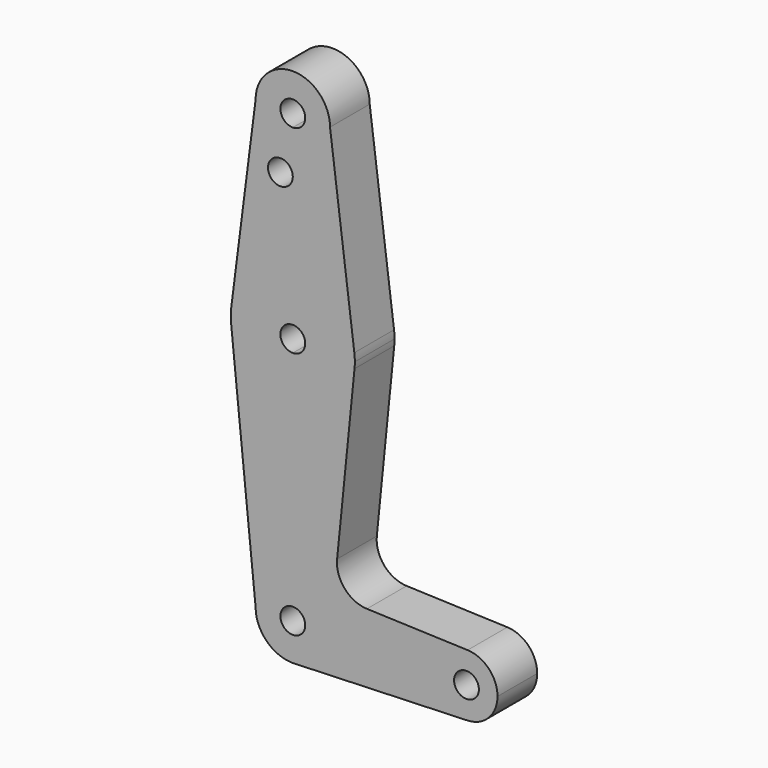
from build123d import *

# Parameters (mm, degrees)
F0_R     = 3.175
F1_DEPTH = 12.7


# Not quite as in the source:
# - a feature names something its author has since deleted; it is built from what else it names


with BuildPart() as f1:
    # F0 (on Front) → F1 (new body)
    with BuildSketch(Plane.XZ):
        with BuildLine():
            Line((0, 9.525), (0, 3.175))
            ThreePointArc((0, 3.175), (2.2450640303, 2.2450640303), (3.175, 0))
            Line((3.175, 0), (9.525, 0))
            ThreePointArc((9.525, 0), (6.7351920908, 6.7351920908), (0, 9.525))
        make_face()
        with BuildLine():
            ThreePointArc((3.175, 0), (-2.2450640303, -2.2450640303), (0, 3.175))
            Line((0, 3.175), (0, 9.525))
            ThreePointArc((0, 9.525), (-6.7351920908, 6.7351920908), (-9.525, 0))
            ThreePointArc((-9.525, 0), (-6.7351920908, -6.7351920908), (0, -9.525))
            Line((0, -9.525), (0.6773435479, -9.500885786))
            ThreePointArc((0.6773435479, -9.500885786), (6.9705567315, -6.4912990883), (9.525, 0))
            Line((9.525, 0), (3.175, 0))
        make_face()
        with BuildLine():
            ThreePointArc((-9.525, 0), (-6.7351920908, 6.7351920908), (0, 9.525))
            Line((0, 9.525), (0, 47.625))
            ThreePointArc((0, 47.625), (-10.644756084, 51.722700101), (-15.7942028036, 61.9003804205))
            Line((-15.7942028036, 61.9003804205), (-9.525, 0))
        make_face()
        with BuildLine():
            Line((0, 47.625), (0, 9.525))
            ThreePointArc((0, 9.525), (6.7351920908, 6.7351920908), (9.525, 0))
            Line((9.525, 0), (36.5125, 0))
            ThreePointArc((36.5125, 0), (38.9384772185, 5.7120069047), (44.7334821429, 7.9324362036))
            Line((44.7334821429, 7.9324362036), (18.9676000005, 8.8532337108))
            ThreePointArc((18.9676000005, 8.8532337108), (13.2611998974, 11.5713591498), (11.3411865923, 17.5933818124))
            Line((11.3411865923, 17.5933818124), (15.7954255641, 61.9125))
            ThreePointArc((15.7954255641, 61.9125), (10.6492737428, 51.7267849017), (0, 47.625))
        make_face()
        with BuildLine():
            Line((36.5125, 0), (9.525, 0))
            ThreePointArc((9.525, 0), (6.9705567315, -6.4912990883), (0.6773435479, -9.500885786))
            Line((0.6773435479, -9.500885786), (44.7324052746, -7.9324746146))
            ThreePointArc((44.7324052746, -7.9324746146), (38.9380895153, -5.7116327839), (36.5125, 0))
        make_face()
        with BuildLine():
            ThreePointArc((44.7334821429, 7.9324362036), (38.9384772185, 5.7120069047), (36.5125, 0))
            ThreePointArc((36.5125, 0), (38.9380895153, -5.7116327839), (44.7324052746, -7.9324746146))
            ThreePointArc((44.7324052746, -7.9324746146), (50.1616327839, -5.5119104847), (52.3875, 0))
            ThreePointArc((52.3875, 0), (50.1620069047, 5.5115227815), (44.7334821429, 7.9324362036))
        make_face()
        with BuildLine():
            ThreePointArc((47.625, 0), (44.45, -3.175), (41.275, 0))
            ThreePointArc((41.275, 0), (44.45, 3.175), (47.625, 0))
        make_face(mode=Mode.SUBTRACT)
        with BuildLine():
            Line((0, 60.325), (0, 47.625))
            ThreePointArc((0, 47.625), (10.6492737428, 51.7267849017), (15.7954255641, 61.9125))
            ThreePointArc((15.7954255641, 61.9125), (15.8550939106, 62.7052534459), (15.875, 63.5))
            ThreePointArc((15.875, 63.5), (15.8430821396, 64.5061676396), (15.7474569047, 65.5082893304))
            ThreePointArc((15.7474569047, 65.5082893304), (10.4912828548, 75.4142187767), (0, 79.375))
            Line((0, 79.375), (0, 66.675))
            ThreePointArc((0, 66.675), (2.2450640303, 65.7450640303), (3.175, 63.5))
            ThreePointArc((3.175, 63.5), (2.2450640303, 61.2549359697), (0, 60.325))
        make_face()
        with BuildLine():
            ThreePointArc((-15.7942028036, 61.9003804205), (-10.644756084, 51.722700101), (0, 47.625))
            Line((0, 47.625), (0, 60.325))
            ThreePointArc((0, 60.325), (-3.175, 63.5), (0, 66.675))
            Line((0, 66.675), (0, 79.375))
            ThreePointArc((0, 79.375), (-10.4912828548, 75.4142187767), (-15.7474569047, 65.5082893304))
            ThreePointArc((-15.7474569047, 65.5082893304), (-15.873667691, 63.7056672947), (-15.7942028036, 61.9003804205))
        make_face()
        with BuildLine():
            Line((0, 100.0252), (0, 79.375))
            ThreePointArc((0, 79.375), (10.4912828548, 75.4142187767), (15.7474569047, 65.5082893304))
            Line((15.7474569047, 65.5082893304), (9.525, 114.3))
            ThreePointArc((9.525, 114.3), (6.7351920908, 107.5648079092), (0, 104.775))
            Line((0, 104.775), (0, 100.0252))
        make_face()
        with BuildLine():
            Line((-9.525, 114.3), (-15.7474569047, 65.5082893304))
            ThreePointArc((-15.7474569047, 65.5082893304), (-10.4912828548, 75.4142187767), (0, 79.375))
            Line((0, 79.375), (0, 100.0252))
            Line((0, 100.0252), (0, 104.775))
            ThreePointArc((0, 104.775), (-6.7351920908, 107.5648079092), (-9.525, 114.3))
        make_face()
        with Locations((-3.175, 100.0252)):
            Circle(F0_R, mode=Mode.SUBTRACT)
        with BuildLine():
            ThreePointArc((9.525, 114.3), (0, 123.825), (-9.525, 114.3))
            ThreePointArc((-9.525, 114.3), (-6.7351920908, 107.5648079092), (0, 104.775))
            ThreePointArc((0, 104.775), (6.7351920908, 107.5648079092), (9.525, 114.3))
        make_face()
        with BuildLine():
            ThreePointArc((3.175, 114.3), (2.2450640303, 112.0549359697), (0, 111.125))
            ThreePointArc((0, 111.125), (-2.2450640303, 116.5450640303), (3.175, 114.3))
        make_face(mode=Mode.SUBTRACT)
    extrude(amount=F1_DEPTH)


solid = f1.part
